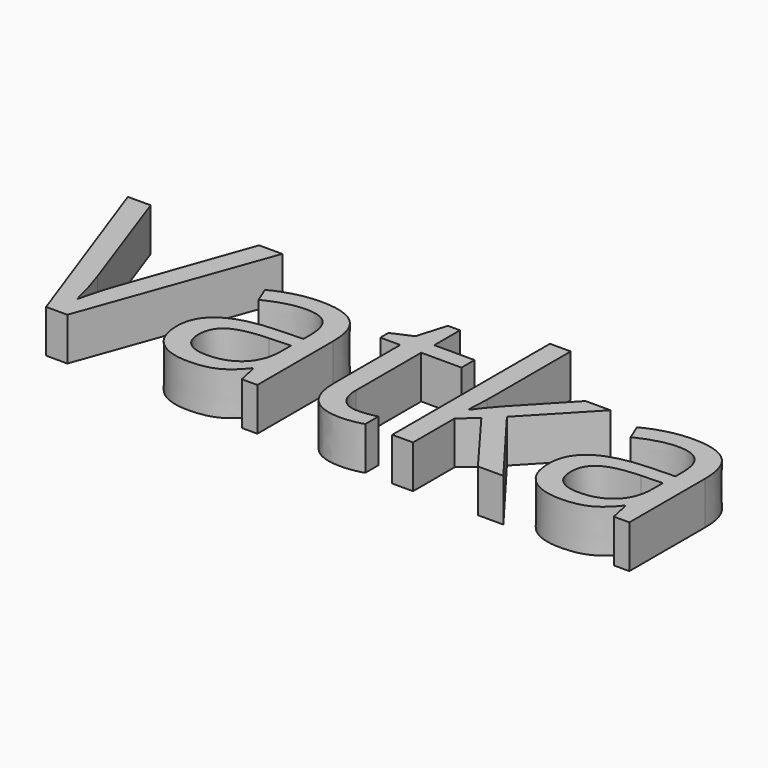
from build123d import *

# Parameters (mm, degrees)
F0_TEXT_SIZE = 76.7135087194
F1_DEPTH     = 12.7


# Not quite as in the source:
# - Text() gives the source's letters only with a copy of the font that has no kerning and outlines rounded to 1/6400 em; it was checked with that copy


with BuildPart() as f1:
    # F0 (on Top) → F1 (new body)
    with BuildSketch(Plane.XY):
        with Locations((-73.6975744367, -20.8310056478)):
            Text('Vatka', F0_TEXT_SIZE, font='Open Sans', text_align=(TextAlign.LEFT, TextAlign.BOTTOM))
    extrude(amount=F1_DEPTH)


solid = f1.part
